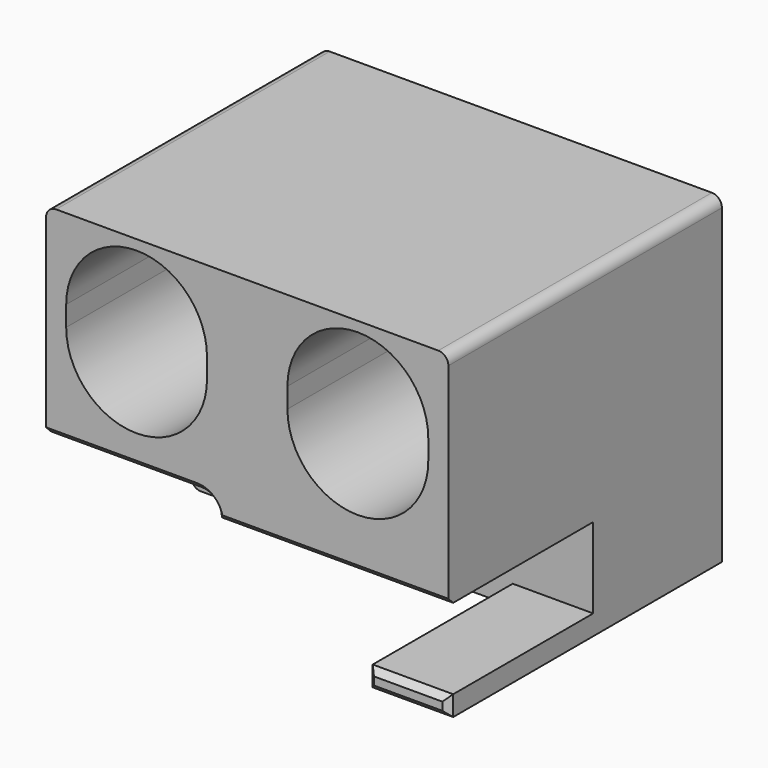
from build123d import *

# Parameters (mm, degrees)
F1_DEPTH = 17
F2_DEPTH = 8
F3_DEPTH = 17
F4_R     = 0.5
F5_DEPTH = 4
F6_SIZE  = 0.3
F7_DEPTH = 7
F8_DEPTH = 4


with BuildPart() as f1:
    # F0 (on Front) → F1 (new body)
    with BuildSketch(Plane.XZ):
        with BuildLine():
            Line((10.7877647579, 0), (10.7877647579, 11))
            Line((10.7877647579, 11), (-9.2122352421, 11))
            Line((-9.2122352421, 11), (-9.2122352421, 1.0579130137))
            ThreePointArc((-9.2122352421, 1.0579130137), (-9.2113932226, 1.0289076607), (-9.2088700001, 1))
            Line((-9.2088700001, 1), (-1.7122352421, 1))
            ThreePointArc((-1.7122352421, 1), (-1.0051284609, 0.7071067812), (-0.7122352421, 0))
            Line((-0.7122352421, 0), (0, 0))
            Line((0, 0), (10.7877647579, 0))
        make_face()
        with BuildLine():
            Line((-8.2122352421, 6), (-8.2122352421, 7))
            ThreePointArc((-8.2122352421, 7), (-4.7122352421, 10.5), (-1.2122352421, 7))
            Line((-1.2122352421, 7), (-1.2122352421, 6))
            ThreePointArc((-1.2122352421, 6), (-4.7122352421, 2.5), (-8.2122352421, 6))
        make_face(mode=Mode.SUBTRACT)
        with BuildLine():
            ThreePointArc((2.7877647579, 7), (6.2877647579, 10.5), (9.7877647579, 7))
            Line((9.7877647579, 7), (9.7877647579, 6))
            ThreePointArc((9.7877647579, 6), (6.2877647579, 2.5), (2.7877647579, 6))
            Line((2.7877647579, 6), (2.7877647579, 7))
        make_face(mode=Mode.SUBTRACT)
    extrude(amount=F1_DEPTH)

    # F0 (on Front) → F2 (join)
    with BuildSketch(Plane.XZ):
        with BuildLine():
            Line((10.7877647579, 0), (10.7877647579, 11))
            Line((10.7877647579, 11), (-9.2122352421, 11))
            Line((-9.2122352421, 11), (-9.2122352421, 1.0579130137))
            ThreePointArc((-9.2122352421, 1.0579130137), (-9.2113932226, 1.0289076607), (-9.2088700001, 1))
            Line((-9.2088700001, 1), (-1.7122352421, 1))
            ThreePointArc((-1.7122352421, 1), (-1.0051284609, 0.7071067812), (-0.7122352421, 0))
            Line((-0.7122352421, 0), (0, 0))
            Line((0, 0), (10.7877647579, 0))
        make_face()
        with BuildLine():
            Line((-8.2122352421, 6), (-8.2122352421, 7))
            ThreePointArc((-8.2122352421, 7), (-4.7122352421, 10.5), (-1.2122352421, 7))
            Line((-1.2122352421, 7), (-1.2122352421, 6))
            ThreePointArc((-1.2122352421, 6), (-4.7122352421, 2.5), (-8.2122352421, 6))
        make_face(mode=Mode.SUBTRACT)
        with BuildLine():
            ThreePointArc((2.7877647579, 7), (6.2877647579, 10.5), (9.7877647579, 7))
            Line((9.7877647579, 7), (9.7877647579, 6))
            ThreePointArc((9.7877647579, 6), (6.2877647579, 2.5), (2.7877647579, 6))
            Line((2.7877647579, 6), (2.7877647579, 7))
        make_face(mode=Mode.SUBTRACT)
        with BuildLine():
            Line((10.7877647579, -4), (10.7877647579, 0))
            Line((10.7877647579, 0), (0, 0))
            Line((0, 0), (-0.7122352421, 0))
            ThreePointArc((-0.7122352421, 0), (-1.0051284609, 0.7071067812), (-1.7122352421, 1))
            Line((-1.7122352421, 1), (-9.2088700001, 1))
            ThreePointArc((-9.2088700001, 1), (-9.2113932226, 1.0289076607), (-9.2122352421, 1.0579130137))
            Line((-9.2122352421, 1.0579130137), (-9.2122352421, -4.5))
            ThreePointArc((-9.2122352421, -4.5), (-9.0657886327, -4.8535533906), (-8.7122352421, -5))
            Line((-8.7122352421, -5), (6.7877647579, -5))
            Line((6.7877647579, -5), (6.7877647579, -4))
            Line((6.7877647579, -4), (10.7877647579, -4))
        make_face()
    extrude(amount=F2_DEPTH)

    # F0 (on Front) → F3 (join)
    with BuildSketch(Plane.XZ):
        with BuildLine():
            Line((10.7877647579, -5), (10.7877647579, -4))
            Line((10.7877647579, -4), (6.7877647579, -4))
            Line((6.7877647579, -4), (6.7877647579, -5))
            Line((6.7877647579, -5), (8.0377647579, -5))
            ThreePointArc((8.0377647579, -5), (8.7877647579, -4.25), (9.5377647579, -5))
            Line((9.5377647579, -5), (10.7877647579, -5))
        make_face()
        with BuildLine():
            Line((8.0377647579, -5), (9.5377647579, -5))
            ThreePointArc((9.5377647579, -5), (8.7877647579, -4.25), (8.0377647579, -5))
        make_face()
    extrude(amount=F3_DEPTH)

    # F4
    f4_edges = [f1.edges().sort_by_distance(p)[0] for p in [
        (-9.212235, -8.5, 11),
        (10.787765, -8.5, 11),
    ]]
    fillet(f4_edges, radius=F4_R)

    # F0 (on Front) → F5 (join)
    with BuildSketch(Plane.XZ):
        with BuildLine():
            Line((9.7877647579, 6), (9.7877647579, 7))
            ThreePointArc((9.7877647579, 7), (6.2877647579, 10.5), (2.7877647579, 7))
            Line((2.7877647579, 7), (2.7877647579, 6))
            ThreePointArc((2.7877647579, 6), (6.2877647579, 2.5), (9.7877647579, 6))
        make_face()
        with BuildLine():
            ThreePointArc((4.2877647579, 7), (6.2877647579, 9), (8.2877647579, 7))
            Line((8.2877647579, 7), (8.2877647579, 6))
            ThreePointArc((8.2877647579, 6), (6.2877647579, 4), (4.2877647579, 6))
            Line((4.2877647579, 6), (4.2877647579, 7))
        make_face(mode=Mode.SUBTRACT)
    extrude(amount=F5_DEPTH)

    # F6
    f6_edges = [f1.edges().sort_by_distance(p)[0] for p in [
        (-5.460553, -17, 1),
        (-1.005128, -17, 0.707107),
        (5.037765, -17, 0),
        (8.787765, -17, -5),
        (6.787765, -17, -4.5),
        (8.787765, -17, -4),
        (10.787765, -17, -4.5),
    ]]
    chamfer(f6_edges, length=F6_SIZE)

    # F0 (on Front) → F7 (cut)
    with BuildSketch(Plane.XZ):
        with BuildLine():
            Line((8.0377647579, -5), (9.5377647579, -5))
            ThreePointArc((9.5377647579, -5), (8.7877647579, -4.25), (8.0377647579, -5))
        make_face()
    extrude(amount=F7_DEPTH, mode=Mode.SUBTRACT)

    # F0 (on Front) → F8 (join)
    with BuildSketch(Plane.XZ):
        with BuildLine():
            ThreePointArc((-1.2122352421, 7), (-4.7122352421, 10.5), (-8.2122352421, 7))
            Line((-8.2122352421, 7), (-8.2122352421, 6))
            ThreePointArc((-8.2122352421, 6), (-4.7122352421, 2.5), (-1.2122352421, 6))
            Line((-1.2122352421, 6), (-1.2122352421, 7))
        make_face()
        with BuildLine():
            Line((-2.7122352421, 7), (-2.7122352421, 6))
            ThreePointArc((-2.7122352421, 6), (-4.7122352421, 4), (-6.7122352421, 6))
            Line((-6.7122352421, 6), (-6.7122352421, 7))
            ThreePointArc((-6.7122352421, 7), (-4.7122352421, 9), (-2.7122352421, 7))
        make_face(mode=Mode.SUBTRACT)
    extrude(amount=F8_DEPTH)


solid = f1.part
